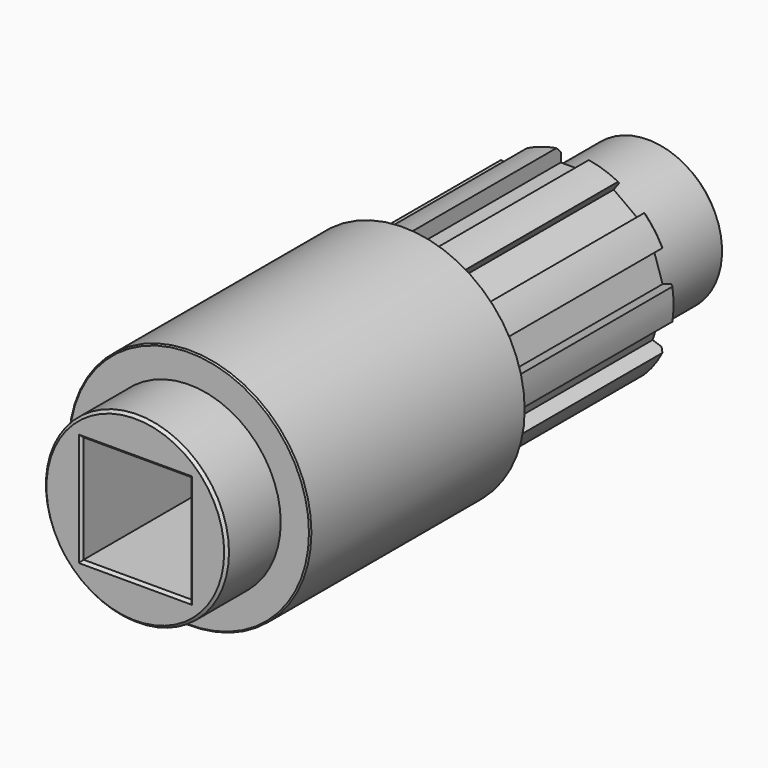
from build123d import *

# Parameters (mm, degrees)
F0_R            = 45
F0_W            = 40
F0_H            = 40
F1_DEPTH        = 100
F2_R            = 34
F2_W            = 40
F2_H            = 40
F3_DEPTH        = 25
F4_R            = 37.5
F5_DEPTH        = 80
F5_DEPTH_BACK   = 50
F6_SIZE         = 2
F7_W            = 12
F7_H            = 15
F8_DEPTH        = 80
F8_COPIES_COUNT = 10
F9_SIZE         = 0.5
F10_R           = 27.5
F11_DEPTH       = 35
F12_SIZE        = 2
F13_SIZE        = 1


# Not quite as in the source:
# - a pattern or mirror of a feature is missing from the dataset's text; its kind, count and spacing are read off the source's solid


with BuildPart() as f1:
    # F0 (on Front) → F1 (new body)
    with BuildSketch(Plane.XZ):
        Circle(F0_R)
        Rectangle(F0_W, F0_H, mode=Mode.SUBTRACT)
    extrude(amount=F1_DEPTH)

    # F2 (on face) → F3 (join)
    with BuildSketch(Plane.XZ.offset(100)):
        Circle(F2_R)
        Rectangle(F2_W, F2_H, mode=Mode.SUBTRACT)
    extrude(amount=F3_DEPTH)

    # F4 (on face) → F5 (join, two sides)
    with BuildSketch(Plane(origin=(0, 0, 0), x_dir=(-1, 0, 0), z_dir=(0, 1, 0))) as f5_sk:
        Circle(F4_R)
    extrude(amount=F5_DEPTH)
    extrude(f5_sk.sketch, amount=-F5_DEPTH_BACK)

    # F6
    f6_edges = [f1.edges().sort_by_distance(p)[0] for p in [
        (37.5, 80, 0),
    ]]
    chamfer(f6_edges, length=F6_SIZE)

    # F7 (on face) → F8 (cut, through all)
    with BuildSketch(Plane(origin=(0, 80, 0), x_dir=(-1, 0, 0), z_dir=(0, 1, 0))):
        with Locations((0, 39)):
            Rectangle(F7_W, F7_H)
    f8 = extrude(amount=-F8_DEPTH, mode=Mode.SUBTRACT)

    # F8_copies: F8 ×10 about axis
    f8_copies_axis = Axis((0, 0, 0), (0, 1, 0))
    for i in range(1, F8_COPIES_COUNT):
        add(f8.rotate(f8_copies_axis, i * 360 / F8_COPIES_COUNT), mode=Mode.SUBTRACT)

    # F9
    f9_edges = [f1.edges().sort_by_distance(p)[0] for p in [
        (45, -50, 0),
        (-45, 0, 0),
        (-45, -100, 0),
    ]]
    chamfer(f9_edges, length=F9_SIZE)

    # F10 (on face) → F11 (join)
    with BuildSketch(Plane(origin=(0, 80, 0), x_dir=(-1, 0, 0), z_dir=(0, 1, 0))):
        Circle(F10_R)
    extrude(amount=F11_DEPTH)

    # F12
    f12_edges = [f1.edges().sort_by_distance(p)[0] for p in [
        (27.5, 115, 0),
    ]]
    chamfer(f12_edges, length=F12_SIZE)

    # F13
    f13_edges = [f1.edges().sort_by_distance(p)[0] for p in [
        (-34, -125, 0),
        (0, -125, 20),
        (20, -125, 0),
        (0, -125, -20),
        (-20, -125, 0),
    ]]
    chamfer(f13_edges, length=F13_SIZE)


solid = f1.part
